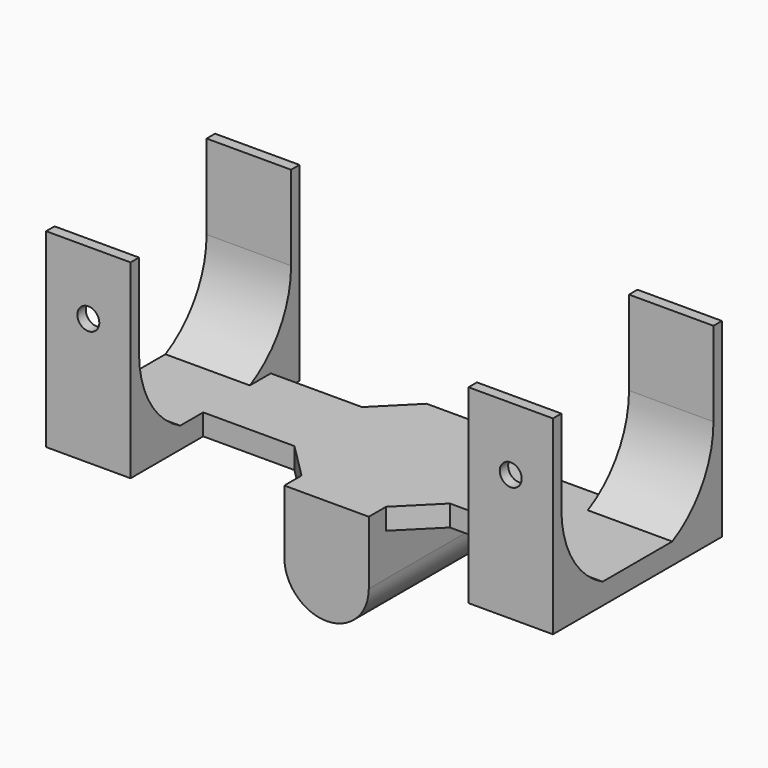
from build123d import *

# Parameters (mm, degrees)
F0_W      = 25
F0_H      = 10
F0_W_2    = 10
F0_H_2    = 4.25
F1_DEPTH  = 2.5
F3_DEPTH  = 2.5
F4_DEPTH  = 18.5
F5_SIZE   = 4.2
F6_W      = 10
F6_H      = 4.25
F6_H_2    = 10
F6_H_3    = 10.75
F7_DEPTH  = 2.5
F8_DEPTH  = 20
F10_DEPTH = 60
F12_DEPTH = 10


with BuildPart() as f1:
    # F0 (on Top) → F1 (new body)
    with BuildSketch(Plane.XY):
        with Locations((-17.5, 0)):
            Rectangle(F0_W, F0_H)
        with Locations((0, 7.125)):
            Rectangle(F0_W_2, F0_H_2)
        Rectangle(F0_W_2, F0_H)
        with Locations((0, -7.125)):
            Rectangle(F0_W_2, F0_H_2)
        with Locations((17.5, 0)):
            Rectangle(F0_W, F0_H)
    extrude(amount=F1_DEPTH)

    # F2 (on face) → F3 (join)
    with BuildSketch(Plane.XZ.offset(9.25)):
        with BuildLine():
            Line((0, 0), (-5, 0))
            Line((-5, 0), (-5, -5))
            ThreePointArc((-5, -5), (-3.5355339059, -1.4644660941), (0, 0))
        make_face()
        with BuildLine():
            Line((5, 0), (0, 0))
            ThreePointArc((0, 0), (3.5355339059, -1.4644660941), (5, -5))
            Line((5, -5), (5, 0))
        make_face()
        with BuildLine():
            ThreePointArc((5, -5), (3.5355339059, -1.4644660941), (0, 0))
            ThreePointArc((0, 0), (-3.5355339059, -1.4644660941), (-5, -5))
            Line((-5, -5), (-2.5, -5))
            ThreePointArc((-2.5, -5), (0, -2.5), (2.5, -5))
            Line((2.5, -5), (5, -5))
        make_face()
        with BuildLine():
            Line((-2.5, -5), (-5, -5))
            ThreePointArc((-5, -5), (0, -10), (5, -5))
            Line((5, -5), (2.5, -5))
            ThreePointArc((2.5, -5), (0, -7.5), (-2.5, -5))
        make_face()
        with BuildLine():
            Line((2.5, -5), (-2.5, -5))
            ThreePointArc((-2.5, -5), (0, -7.5), (2.5, -5))
        make_face()
        with BuildLine():
            ThreePointArc((2.5, -5), (0, -2.5), (-2.5, -5))
            Line((-2.5, -5), (2.5, -5))
        make_face()
        Polygon((-5, 2.5), (-5, 0), (0, 0), (5, 0), (5, 2.5), align=None)
    extrude(amount=F3_DEPTH)

    # F2 (on face) → F4 (join)
    with BuildSketch(Plane.XZ.offset(9.25)):
        with BuildLine():
            ThreePointArc((5, -5), (3.5355339059, -1.4644660941), (0, 0))
            ThreePointArc((0, 0), (-3.5355339059, -1.4644660941), (-5, -5))
            Line((-5, -5), (-2.5, -5))
            ThreePointArc((-2.5, -5), (0, -2.5), (2.5, -5))
            Line((2.5, -5), (5, -5))
        make_face()
        with BuildLine():
            Line((-2.5, -5), (-5, -5))
            ThreePointArc((-5, -5), (0, -10), (5, -5))
            Line((5, -5), (2.5, -5))
            ThreePointArc((2.5, -5), (0, -7.5), (-2.5, -5))
        make_face()
        with BuildLine():
            Line((0, 0), (-5, 0))
            Line((-5, 0), (-5, -5))
            ThreePointArc((-5, -5), (-3.5355339059, -1.4644660941), (0, 0))
        make_face()
        with BuildLine():
            Line((5, 0), (0, 0))
            ThreePointArc((0, 0), (3.5355339059, -1.4644660941), (5, -5))
            Line((5, -5), (5, 0))
        make_face()
    extrude(amount=-F4_DEPTH)

    # F5
    f5_edges = [f1.edges().sort_by_distance(p)[0] for p in [
        (-5, 5, 1.25),
        (-5, -5, 1.25),
        (5, 5, 1.25),
        (5, -5, 1.25),
    ]]
    chamfer(f5_edges, length=F5_SIZE)

    # F6 (on face) → F7 (join)
    with BuildSketch(Plane.XY.offset(2.5)):
        with Locations((-25, 7.125)):
            Rectangle(F6_W, F6_H)
        with Locations((-25, 0)):
            Rectangle(F6_W, F6_H_2)
        with Locations((-25, -10.375)):
            Rectangle(F6_W, F6_H_3)
        with Locations((25, 7.125)):
            Rectangle(F6_W, F6_H)
        with Locations((25, 0)):
            Rectangle(F6_W, F6_H_2)
        with Locations((25, -10.375)):
            Rectangle(F6_W, F6_H_3)
    extrude(amount=-F7_DEPTH)

    # F6 (on face) → F8 (join)
    with BuildSketch(Plane.XY.offset(2.5)):
        with Locations((-25, 7.125)):
            Rectangle(F6_W, F6_H)
        with Locations((-25, 0)):
            Rectangle(F6_W, F6_H_2)
        with Locations((-25, -10.375)):
            Rectangle(F6_W, F6_H_3)
        with Locations((25, -10.375)):
            Rectangle(F6_W, F6_H_3)
        with Locations((25, 0)):
            Rectangle(F6_W, F6_H_2)
        with Locations((25, 7.125)):
            Rectangle(F6_W, F6_H)
    extrude(amount=F8_DEPTH)

    # F9 (on face) → F10 (cut)
    with BuildSketch(Plane(origin=(-30, 0, 0), x_dir=(0, -1, 0), z_dir=(-1, 0, 0))):
        with BuildLine():
            ThreePointArc((8.403882032, 2.5), (12.855823048, 6.644176952), (14.5, 12.5))
            ThreePointArc((14.5, 12.5), (12.855823048, 18.355823048), (8.403882032, 22.5))
            Line((8.403882032, 22.5), (3.25, 22.5))
            Line((3.25, 22.5), (-1.903882032, 22.5))
            ThreePointArc((-1.903882032, 22.5), (-6.355823048, 18.355823048), (-8, 12.5))
            ThreePointArc((-8, 12.5), (-6.355823048, 6.644176952), (-1.903882032, 2.5))
            Line((-1.903882032, 2.5), (8.403882032, 2.5))
        make_face()
        with BuildLine():
            ThreePointArc((8.403882032, 22.5), (12.855823048, 18.355823048), (14.5, 12.5))
            Line((14.5, 12.5), (14.5, 22.5))
            Line((14.5, 22.5), (8.403882032, 22.5))
        make_face()
        with BuildLine():
            ThreePointArc((-8, 12.5), (-6.355823048, 18.355823048), (-1.903882032, 22.5))
            Line((-1.903882032, 22.5), (-8, 22.5))
            Line((-8, 22.5), (-8, 12.5))
        make_face()
    extrude(amount=-F10_DEPTH, mode=Mode.SUBTRACT)

    # F11 (on face) → F12 (cut)
    with BuildSketch(Plane.XZ.offset(15.75)):
        with BuildLine():
            Line((-25, 15), (-25, 16.3))
            ThreePointArc((-25, 16.3), (-25.9192388155, 14.0807611845), (-23.7, 15))
            Line((-23.7, 15), (-25, 15))
        make_face()
        with BuildLine():
            ThreePointArc((-23.7, 15), (-24.0807611845, 15.9192388155), (-25, 16.3))
            Line((-25, 16.3), (-25, 15))
            Line((-25, 15), (-23.7, 15))
        make_face()
        with BuildLine():
            ThreePointArc((26.3, 15), (25, 16.3), (23.7, 15))
            ThreePointArc((23.7, 15), (25, 13.7), (26.3, 15))
        make_face()
    extrude(amount=-F12_DEPTH, mode=Mode.SUBTRACT)


solid = f1.part
